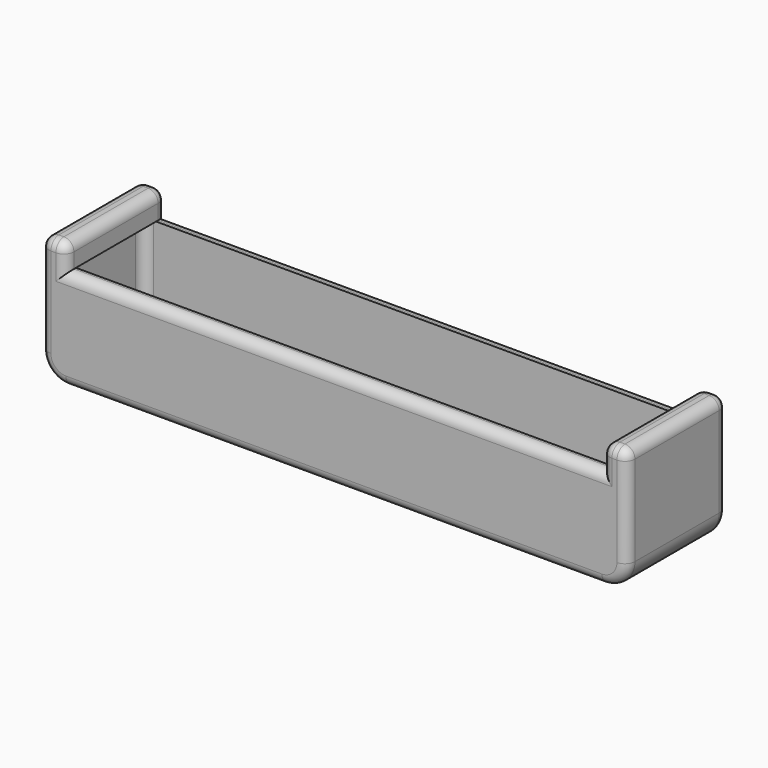
from build123d import *

# Parameters (mm, degrees)
F1_DEPTH     = 25
F2_T         = -2.5
F3_R         = 2
F4_T1_DEPTH  = 25
F4_T4_ANGLE  = 90
F4_T6_ANGLE  = 90
F4_T8_ANGLE  = 90
F4_T10_ANGLE = 90


# Not quite as in the source:
# - a fillet or chamfer that OpenCascade refuses, or shapes differently, is made with other operations: its cross-section is extruded or revolved along the edge and cut away or added
# - a shell that OpenCascade refuses in one call is made with other operations: the cavity is built on its own and cut out


with BuildPart() as f1:
    # F0 (on Front) → F1 (new body)
    with BuildSketch(Plane.XZ):
        Polygon((67.4263688624, 0), (-39.5736311376, 0), (-39.5736311376, 5), (-44.5736311376, 5), (-44.5736311376, -20), (72.4263688624, -20), (72.4263688624, 5), (67.4263688624, 5), align=None)
    extrude(amount=F1_DEPTH)

    # F2: a shell. OpenCascade refuses it in one call, so the cavity is built on its own and cut out:
    # the body offset inwards by the wall thickness, plus a prism from it out through each open face.
    f2_core = offset(f1.part, amount=F2_T, kind=Kind.INTERSECTION, mode=Mode.PRIVATE)
    f2_exits = [f2_core.faces().sort_by_distance(p)[0] for p in [
        (13.926369, -12.5, -2.5),
    ]]
    add(f2_core, mode=Mode.SUBTRACT)
    extrude(f2_exits, amount=-F2_T, mode=Mode.SUBTRACT)

    # F3
    f3_edges = [f1.edges().sort_by_distance(p)[0] for p in [
        (-39.573631, -12.5, 5),
        (-44.573631, -12.5, 5),
        (-42.073631, 0, 5),
        (-42.073631, -25, 5),
        (13.926369, -25, 0),
        (-39.573631, -25, 2.5),
        (-44.573631, -25, -7.5),
        (13.926369, -25, -20),
        (72.426369, -25, -7.5),
        (69.926369, -25, 5),
        (67.426369, -25, 2.5),
        (13.926369, 0, 0),
        (-39.573631, 0, 2.5),
        (-44.573631, 0, -7.5),
        (13.926369, 0, -20),
        (72.426369, 0, -7.5),
        (69.926369, 0, 5),
        (67.426369, 0, 2.5),
        (13.926369, -2.5, -17.5),
        (69.926369, -12.5, -17.5),
        (13.926369, -22.5, -17.5),
        (-42.073631, -12.5, -17.5),
        (-42.073631, -22.5, -8.75),
        (-42.073631, -12.5, 0),
        (-42.073631, -2.5, -8.75),
        (69.926369, -12.5, 0),
        (69.926369, -22.5, -8.75),
        (69.926369, -2.5, -8.75),
        (72.426369, -12.5, 5),
        (67.426369, -12.5, 5),
    ]]
    fillet(f3_edges, radius=F3_R)

    # F4: fillet of radius 5 on 2 edges, made by hand

    # F4_s2 → F4_t1 (cut)
    with BuildSketch(Plane.XZ):
        with BuildLine():
            ThreePointArc((67.4263688624, -20), (70.9619027683, -18.5355339059), (72.4263688624, -15))
            Line((72.4263688624, -15), (72.4263688624, -20))
            Line((72.4263688624, -20), (67.4263688624, -20))
        make_face()
        with BuildLine():
            ThreePointArc((-44.5736311376, -15), (-43.1091650435, -18.5355339059), (-39.5736311376, -20))
            Line((-39.5736311376, -20), (-44.5736311376, -20))
            Line((-44.5736311376, -20), (-44.5736311376, -15))
        make_face()
    extrude(amount=F4_T1_DEPTH, mode=Mode.SUBTRACT)

    # F4_s3 → F4_t4 (revolve, cut)
    with BuildSketch(Plane.YZ.offset(-39.5736311376)):
        with BuildLine():
            ThreePointArc((0, -18), (-0.5857864376, -19.4142135624), (-2, -20))
            Line((-2, -20), (0, -20))
            Line((0, -20), (0, -18))
        make_face()
    revolve(axis=Axis((-39.5736311376, 0, -15), (0, 1, 0)), revolution_arc=F4_T4_ANGLE, mode=Mode.SUBTRACT)

    # F4_s5 → F4_t6 (revolve, cut)
    with BuildSketch(Plane.XY.offset(-15)):
        with BuildLine():
            ThreePointArc((-42.5736311376, -25), (-43.9878447, -24.4142135624), (-44.5736311376, -23))
            Line((-44.5736311376, -23), (-44.5736311376, -25))
            Line((-44.5736311376, -25), (-42.5736311376, -25))
        make_face()
    revolve(axis=Axis((-39.5736311376, -25, -15), (0, -1, 0)), revolution_arc=F4_T6_ANGLE, mode=Mode.SUBTRACT)

    # F4_s7 → F4_t8 (revolve, cut)
    with BuildSketch(Plane.XY.offset(-15)):
        with BuildLine():
            ThreePointArc((70.4263688624, 0), (71.8405824248, -0.5857864376), (72.4263688624, -2))
            Line((72.4263688624, -2), (72.4263688624, 0))
            Line((72.4263688624, 0), (70.4263688624, 0))
        make_face()
    revolve(axis=Axis((67.4263688624, 0, -15), (0, 1, 0)), revolution_arc=F4_T8_ANGLE, mode=Mode.SUBTRACT)

    # F4_s9 → F4_t10 (revolve, cut)
    with BuildSketch(Plane.YZ.offset(67.4263688624)):
        with BuildLine():
            ThreePointArc((-25, -18), (-24.4142135624, -19.4142135624), (-23, -20))
            Line((-23, -20), (-25, -20))
            Line((-25, -20), (-25, -18))
        make_face()
    revolve(axis=Axis((67.4263688624, -25, -15), (0, -1, 0)), revolution_arc=F4_T10_ANGLE, mode=Mode.SUBTRACT)


solid = f1.part
